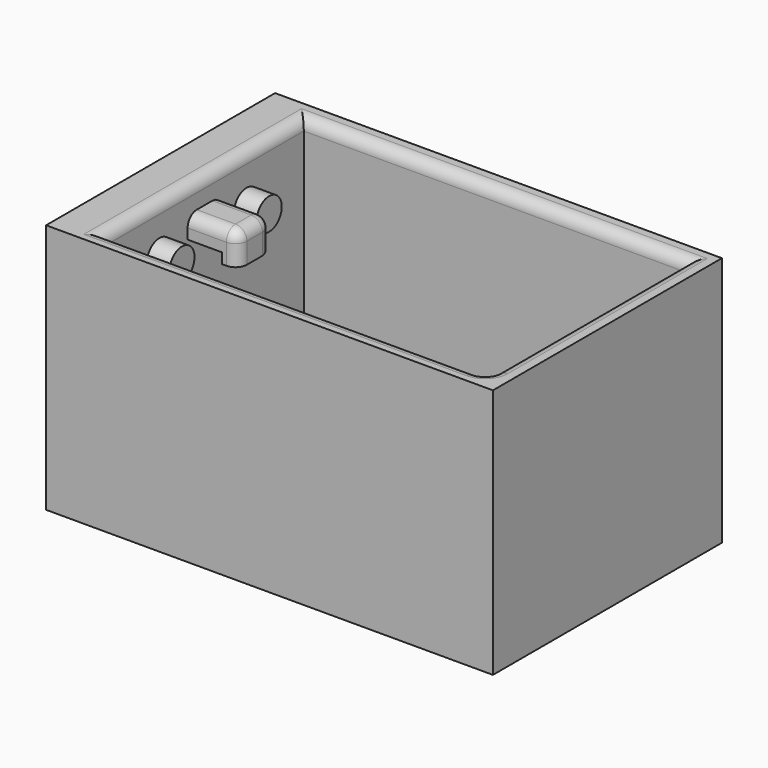
from build123d import *

# Parameters (mm, degrees)
F0_W      = 196.0822343826
F0_H      = 109.9328920245
F1_DEPTH  = 62.8
F2_W      = 168.0704802275
F2_H      = 109.4043701887
F3_DEPTH  = 95
F4_R      = 6.9163922732
F5_DEPTH  = 8.9
F6_W      = 18.5355395079
F6_H      = 9.5271170139
F7_DEPTH  = 22
F8_W      = 6.9370792508
F8_H      = 18.5355395079
F9_DEPTH  = 14.1
F10_R     = 5
F11_R     = 6.8989817164
F11_R_2   = 6.9010656104
F12_DEPTH = 9.9


with BuildPart() as f1:
    # F0 (on Front) → F1 (new body, symmetric)
    with BuildSketch(Plane.XZ):
        Rectangle(F0_W, F0_H)
    extrude(amount=F1_DEPTH, both=True)

    # F2 (on face) → F3 (cut)
    with BuildSketch(Plane.XY.offset(54.9664460123)):
        with Locations((5.2852407098, -0.2642609179)):
            Rectangle(F2_W, F2_H)
    extrude(amount=-F3_DEPTH, mode=Mode.SUBTRACT)

    # F4 (on face) → F5 (cut)
    with BuildSketch(Plane.XY.offset(-40.0335539877)):
        with Locations((-64.4798651338, 0)):
            Circle(F4_R)
    extrude(amount=-F5_DEPTH, mode=Mode.SUBTRACT)

    # F6 (on face) → F7 (join)
    with BuildSketch(Plane.YZ.offset(-78.749999404)):
        with Locations((0, 38.6865362525)):
            Rectangle(F6_W, F6_H)
    extrude(amount=F7_DEPTH)

    # F8 (on face) → F9 (join)
    with BuildSketch(Plane.XY.offset(43.4500947595)):
        with Locations((-60.2185390294, 0)):
            Rectangle(F8_W, F8_H)
    extrude(amount=-F9_DEPTH)

    # F10
    f10_edges = [f1.edges().sort_by_distance(p)[0] for p in [
        (5.285241, -54.966446, 54.966446),
        (89.320481, -54.966446, 7.466446),
        (5.285241, -54.966446, -40.033554),
        (-67.749999, 9.26777, 43.450095),
        (-67.749999, -9.26777, 43.450095),
        (-56.749999, 0, 43.450095),
        (-60.218539, 9.26777, 29.350095),
        (-56.749999, -9.26777, 36.400095),
        (-78.749999, -0.264261, 54.966446),
        (5.285241, 54.437924, 54.966446),
        (-78.749999, -0.264261, -40.033554),
        (5.285241, 54.437924, -40.033554),
        (89.320481, -0.264261, -40.033554),
        (-56.749999, 9.26777, 36.400095),
        (89.320481, -0.264261, 54.966446),
    ]]
    fillet(f10_edges, radius=F10_R)

    # F11 (on face) → F12 (join)
    with BuildSketch(Plane.YZ.offset(-78.749999404)):
        with Locations((-24.7665680945, 33.9229777455)):
            Circle(F11_R)
        with Locations((23.0645500124, 33.9229777455)):
            Circle(F11_R_2)
    extrude(amount=F12_DEPTH)


solid = f1.part
